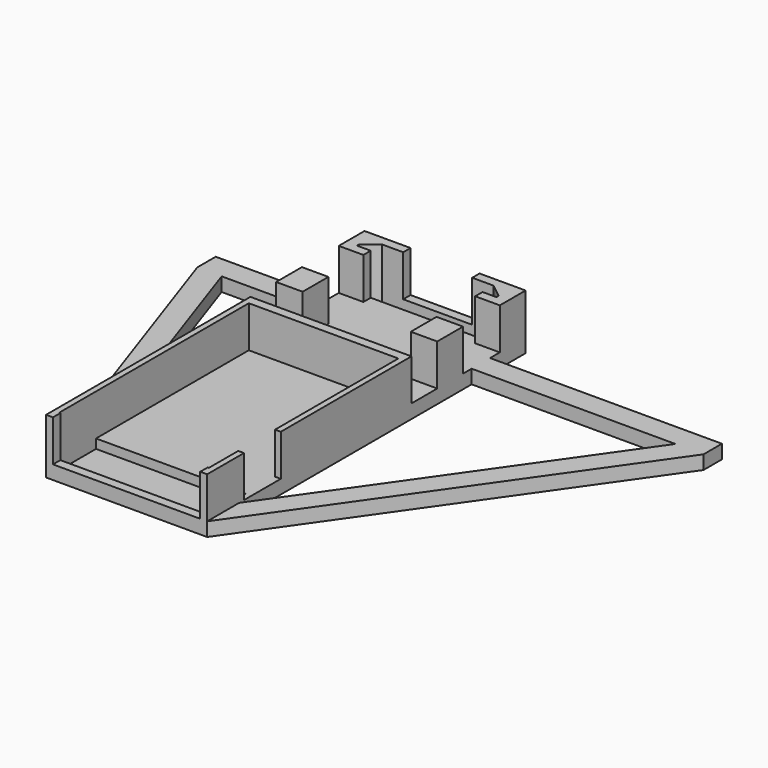
from build123d import *

# Parameters (mm, degrees)
F0_W     = 5
F0_H     = 5
F0_W_2   = 5.75
F0_H_2   = 7
F1_DEPTH = 3
F2_DEPTH = 1
F3_DEPTH = 12


# Not quite as in the source:
# - a feature names something its author has since deleted; it is built from what else it names


with BuildPart() as f1:
    # F0 (on Top) → F1 (new body)
    with BuildSketch(Plane.XY):
        Polygon((-7.5, 41.25), (-7.5, 43.25), (-17.5, 43.25), (-17.5, 36.25), (-12.15, 36.25), (-12.15, 38.25), (-15.15, 38.25), (-15.15, 38.85), (-12.15, 41.25), align=None)
        Polygon((7.5, 43.25), (0, 43.25), (-7.5, 43.25), (-7.5, 41.25), (0, 41.25), (7.5, 41.25), align=None)
        Polygon((17.5, 43.25), (7.5, 43.25), (7.5, 41.25), (12.15, 41.25), (15.15, 38.85), (15.15, 38.25), (12.15, 38.25), (12.15, 36.25), (17.5, 36.25), align=None)
        Polygon((-17.5, 0), (-17.5, -27.8208897438), (-17.5, -43.25), (-16, -43.25), (-16, -41.25), (-16.25, -41.25), (-16.25, -31.25), (-16.25, 10.25), (0, 10.25), (16.25, 10.25), (16.25, -23.25), (17.5, -23.25), (17.5, 0), (17.5, 12.25), (-17.5, 12.25), align=None)
        Polygon((16.25, -33.25), (17.5, -33.25), (17.5, -23.25), (16.25, -23.25), (16.25, -31.25), align=None)
        Polygon((62.8901566565, 28.5934534669), (61.7828955537, 28.5934534669), (17.5, -34.5426103437), (17.5, -43.25), (67.8901566565, 28.5934534669), align=None)
        Polygon((-17.5, 28.5934534669), (-17.5, 33.5934534669), (-37.1098433435, 33.5934534669), (-37.1098433435, 28.5934534669), (-36.8246298966, 28.5934534669), align=None)
        with Locations((-39.6098433435, 31.0934534669)):
            Rectangle(F0_W, F0_H)
        with Locations((65.3901566565, 31.0934534669)):
            Rectangle(F0_W, F0_H)
        Polygon((62.8901566565, 33.5934534669), (17.5, 33.5934534669), (17.5, 28.5934534669), (61.7828955537, 28.5934534669), (62.8901566565, 28.5934534669), align=None)
        Polygon((16.25, -31.25), (16.25, -23.25), (16.25, 10.25), (0, 10.25), (-16.25, 10.25), (-16.25, -31.25), align=None)
        Polygon((-17.5, -27.8208897438), (-36.8246298966, 28.5934534669), (-37.1098433435, 28.5934534669), (-42.1098433435, 28.5934534669), (-17.5, -43.25), align=None)
        Polygon((-16, -41.25), (-16, -43.25), (0, -43.25), (16, -43.25), (16, -41.25), (0, -41.25), align=None)
        Polygon((17.5, -43.25), (17.5, -34.5426103437), (17.5, -33.25), (16.25, -33.25), (16.25, -41.25), (16, -41.25), (16, -43.25), align=None)
        Polygon((-12.15, 36.25), (-17.5, 36.25), (-17.5, 33.5934534669), (-17.5, 28.5934534669), (-17.5, 26.25), (-11.75, 26.25), (-11.75, 19.25), (-17.5, 19.25), (-17.5, 12.25), (17.5, 12.25), (17.5, 19.25), (11.75, 19.25), (11.75, 26.25), (17.5, 26.25), (17.5, 28.5934534669), (17.5, 33.5934534669), (17.5, 36.25), (12.15, 36.25), (12.15, 38.25), (0, 38.25), (-12.15, 38.25), align=None)
        with Locations((-14.625, 22.75)):
            Rectangle(F0_W_2, F0_H_2)
        with Locations((14.625, 22.75)):
            Rectangle(F0_W_2, F0_H_2)
    extrude(amount=F1_DEPTH)

    # F0 (on Top) → F2 (join)
    with BuildSketch(Plane.XY):
        Polygon((16.25, -41.25), (16.25, -33.25), (16.25, -31.25), (-16.25, -31.25), (-16.25, -41.25), (-16, -41.25), (0, -41.25), (16, -41.25), align=None)
    extrude(amount=F2_DEPTH)

    # F0 (on Top) → F3 (join)
    with BuildSketch(Plane.XY):
        Polygon((-7.5, 41.25), (-7.5, 43.25), (-17.5, 43.25), (-17.5, 36.25), (-12.15, 36.25), (-12.15, 38.25), (-15.15, 38.25), (-15.15, 38.85), (-12.15, 41.25), align=None)
        Polygon((17.5, 43.25), (7.5, 43.25), (7.5, 41.25), (12.15, 41.25), (15.15, 38.85), (15.15, 38.25), (12.15, 38.25), (12.15, 36.25), (17.5, 36.25), align=None)
        Polygon((-17.5, 0), (-17.5, -27.8208897438), (-17.5, -43.25), (-16, -43.25), (-16, -41.25), (-16.25, -41.25), (-16.25, -31.25), (-16.25, 10.25), (0, 10.25), (16.25, 10.25), (16.25, -23.25), (17.5, -23.25), (17.5, 0), (17.5, 12.25), (-17.5, 12.25), align=None)
        Polygon((17.5, -43.25), (17.5, -34.5426103437), (17.5, -33.25), (16.25, -33.25), (16.25, -41.25), (16, -41.25), (16, -43.25), align=None)
        with Locations((-14.625, 22.75)):
            Rectangle(F0_W_2, F0_H_2)
        with Locations((14.625, 22.75)):
            Rectangle(F0_W_2, F0_H_2)
    extrude(amount=F3_DEPTH)


solid = f1.part
